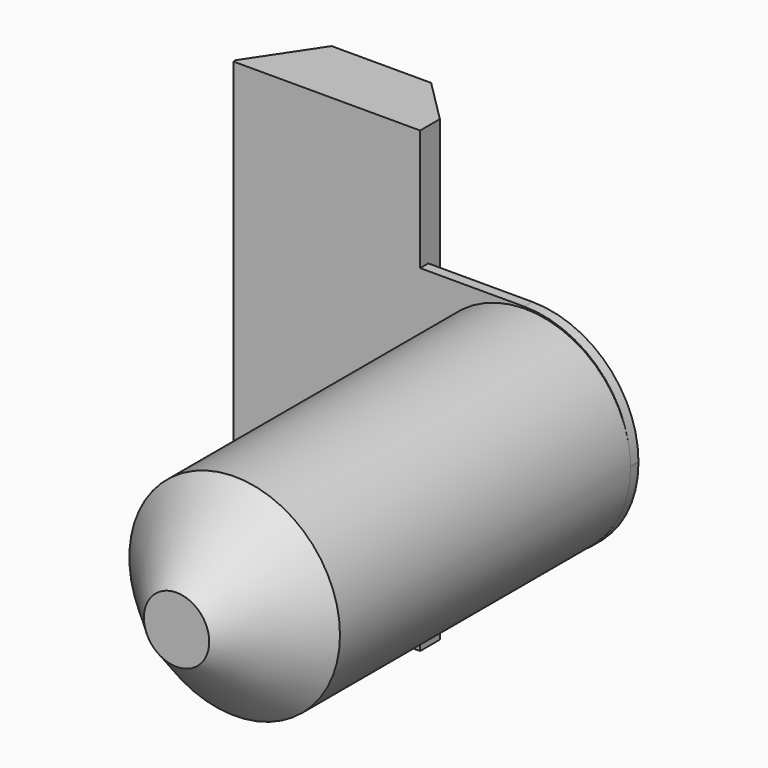
from build123d import *

# Parameters (mm, degrees)
F0_R        = 7.25
F1_DEPTH    = 30
F3_DEPTH    = 4.7
F4_T1_DEPTH = 22.95
F4_T3_DEPTH = 23.089756942
F5_SIZE2    = 4
F5_SIZE     = 5
F6_SIZE2    = 3
F6_SIZE     = 4.5
F7_SIZE     = 5
F8_SIZE     = 3


# Not quite as in the source:
# - a fillet or chamfer that OpenCascade refuses, or shapes differently, is made with other operations: its cross-section is extruded or revolved along the edge and cut away or added


with BuildPart() as f1:
    # F0 (on Front) → F1 (new body)
    with BuildSketch(Plane.XZ):
        Circle(F0_R)
    extrude(amount=F1_DEPTH)

    # F2 (on face) → F3 (join)
    with BuildSketch(Plane(origin=(0, 0, 0), x_dir=(-1, 0, 0), z_dir=(0, 1, 0))):
        Polygon((20.0881361961, 7.1568624116), (7.2347377427, 7.3653035797), (-7.2347377427, 7.3653035797), (-7.2347377427, -7.3653035797), (7.2347377427, -7.2549186188), (20.0881361961, -7.1568624116), align=None)
        Polygon((7.2347377427, 15.7034024596), (7.2347377427, 7.3653035797), (20.0881361961, 7.1568624116), (20.0881361961, 15.7034024596), align=None)
        Polygon((20.0881361961, -15.8427814022), (20.0881361961, -7.1568624116), (7.2347377427, -7.2549186188), (7.2347377427, -15.8427814022), align=None)
    extrude(amount=F3_DEPTH)

    # F4: fillet of radius 7.3 on 2 edges, made by hand

    # F4_s2 → F4_t1 (cut)
    with BuildSketch(Plane.XZ.offset(-22.95)):
        with BuildLine():
            ThreePointArc((7.2347377427, 0.0653035797), (5.0966172454, 5.2271830824), (-0.0652622573, 7.3653035797))
            Line((-0.0652622573, 7.3653035797), (7.2347377427, 7.3653035797))
            Line((7.2347377427, 7.3653035797), (7.2347377427, 0.0653035797))
        make_face()
    extrude(amount=F4_T1_DEPTH, mode=Mode.SUBTRACT)

    # F4_s4 → F4_t3 (cut)
    with BuildSketch(Plane.XZ.offset(-23.089756942)):
        with BuildLine():
            ThreePointArc((7.2347377427, -0.0094008029), (5.0768906111, -5.190931839), (-0.120950991, -7.3091883865))
            Line((-0.120950991, -7.3091883865), (7.2347377427, -7.3653035797))
            Line((7.2347377427, -7.3653035797), (7.2347377427, -0.0094008029))
        make_face()
    extrude(amount=F4_T3_DEPTH, mode=Mode.SUBTRACT)

    # F5
    f5_edges = [f1.edges().sort_by_distance(p)[0] for p in [
        (5.096617, 4.7, 5.227183),
        (5.076891, 4.7, -5.190932),
    ]]
    chamfer(f5_edges, length=F5_SIZE, length2=F5_SIZE2)

    # F6
    f6_edges = [f1.edges().sort_by_distance(p)[0] for p in [
        (-20.088136, 4.7, -0.069689),
    ]]
    f6_side = f1.faces().sort_by_distance((-20.088136, 2.35, -0.069689))[0]
    chamfer(f6_edges, length=F6_SIZE, length2=F6_SIZE2, reference=f6_side)

    # F7
    f7_edges = [f1.edges().sort_by_distance(p)[0] for p in [
        (-7.25, -30, 0),
    ]]
    chamfer(f7_edges, length=F7_SIZE)

    # F8
    f8_edges = [f1.edges().sort_by_distance(p)[0] for p in [
        (-7.234738, 4.7, 11.534353),
        (-7.234738, 4.7, -11.54885),
    ]]
    chamfer(f8_edges, length=F8_SIZE)


solid = f1.part
